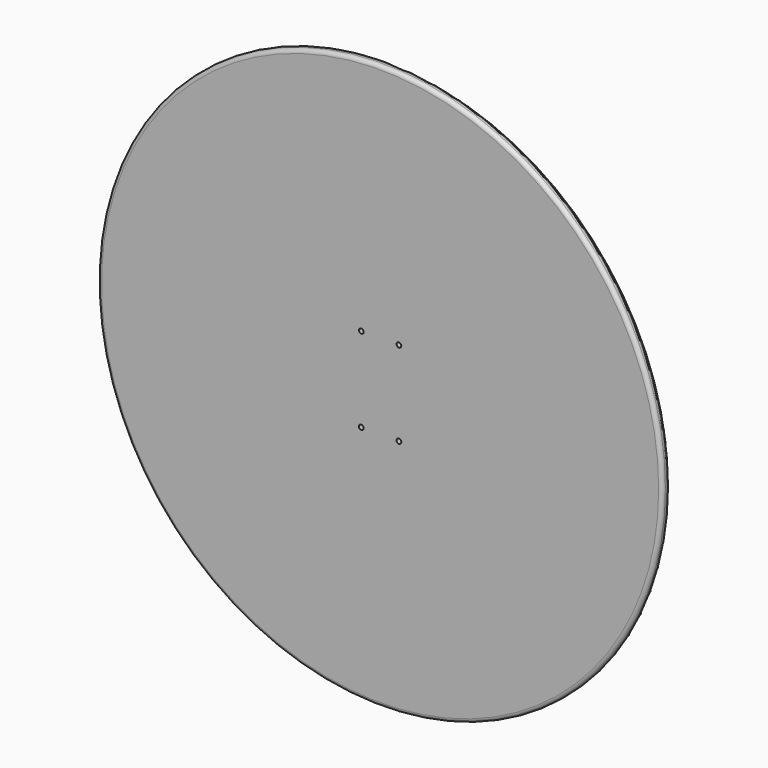
from build123d import *

# Parameters (mm, degrees)
F0_R     = 381
F1_DEPTH = 12.7
F2_R     = 5.08
F3_R     = 3.175
F4_DEPTH = 12.7
F5_R     = 375.92
F6_DEPTH = 2.54
F7_R     = 1.26999
F8_R     = 88.9
F8_R_2   = 50.8
F8_R_3   = 76.2
F9_DEPTH = 12.7
F10_R    = 6.34999


# Not quite as in the source:
# - a fillet or chamfer is up to 0.001 mm smaller than in the source, because OpenCascade refuses the exact size


with BuildPart() as f1:
    # F0 (on Front) → F1 (new body)
    with BuildSketch(Plane.XZ):
        Circle(F0_R)
    extrude(amount=F1_DEPTH)

    # F2
    f2_edges = [f1.edges().sort_by_distance(p)[0] for p in [
        (-381, -12.7, 0),
        (-381, 0, 0),
    ]]
    fillet(f2_edges, radius=F2_R)

    # F3 (on face) → F4 (cut)
    with BuildSketch(Plane.XZ.offset(12.7)):
        with Locations((-25.4, 57.15)):
            Circle(F3_R)
        with Locations((25.4, 57.15)):
            Circle(F3_R)
        with Locations((-25.4, -57.15)):
            Circle(F3_R)
        with Locations((25.4, -57.15)):
            Circle(F3_R)
    extrude(amount=-F4_DEPTH, mode=Mode.SUBTRACT)

    # F5 (on face) → F6 (join)
    with BuildSketch(Plane(origin=(0, 0, 0), x_dir=(-1, 0, 0), z_dir=(0, 1, 0))):
        Circle(F5_R)
        with BuildLine():
            ThreePointArc((13.8301810917, 323.3988637204), (233.7251076258, 223.943459449), (323.6944530953, 0))
            ThreePointArc((323.6944530953, 0), (228.8865428162, -228.8865428162), (0, -323.6944530953))
            ThreePointArc((0, -323.6944530953), (-297.0398470602, -128.6290333601), (-236.0741621082, 221.4657737656))
            ThreePointArc((-236.0741621082, 221.4657737656), (-122.2525479548, 299.7205589933), (13.8301810917, 323.3988637204))
        make_face(mode=Mode.SUBTRACT)
        Polygon((-154.4742758485, 183.9868239484), (-236.0741621082, 221.4657737656), (-282.388240099, -93.3703109622), (-140.2126329417, -183.4818201537), (-33.9375066037, -289.7569464917), align=None)
        with BuildLine():
            ThreePointArc((-236.0741621082, 221.4657737656), (-297.0398470602, -128.6290333601), (0, -323.6944530953))
            Line((0, -323.6944530953), (-33.9375066037, -289.7569464917))
            Line((-33.9375066037, -289.7569464917), (-140.2126329417, -183.4818201537))
            Line((-140.2126329417, -183.4818201537), (-282.388240099, -93.3703109622))
            Line((-282.388240099, -93.3703109622), (-236.0741621082, 221.4657737656))
        make_face()
    extrude(amount=F6_DEPTH)

    # F7 (radius 1.27 in the source; OpenCascade refuses exactly that, so slightly less here)
    f7_edges = [f1.edges().sort_by_distance(p)[0] for p in [
        (94.205891, 2.54, -52.885061),
        (-297.039847, 0, 128.629033),
        (195.274219, 0, 202.726299),
        (94.205891, 0, -52.885061),
        (16.968753, 0, -306.7257),
        (-28.575, 0, -57.15),
        (22.225, 0, -57.15),
        (-28.575, 0, 57.15),
        (22.225, 0, 57.15),
    ]]
    fillet(f7_edges, radius=F7_R)

    # F8 (on face) → F9 (join)
    with BuildSketch(Plane(origin=(0, 0, 0), x_dir=(-1, 0, 0), z_dir=(0, 1, 0))):
        with Locations((-223.9369153976, -103.2387167215)):
            Circle(F8_R)
        with Locations((236.2960875034, 19.1194508225)):
            Circle(F8_R_2)
        with Locations((154.5488387346, -124.6951445937)):
            Circle(F8_R_3)
        Polygon((100.0506654382, 276.4718830585), (-60.4161508381, 225.0014096498), (-110.3727966547, 97.8390201926), (0, 168.989405036), (133.3551108837, 75.1314535737), (196.9362944365, 196.2384879589), (50.0940196216, 175.044760108), align=None)
    extrude(amount=F9_DEPTH)

    # F10 (radius 6.35 in the source; OpenCascade refuses exactly that, so slightly less here)
    f10_edges = [f1.edges().sort_by_distance(p)[0] for p in [
        (-66.677555, 12.7, 122.060429),
        (-165.145703, 12.7, 135.684971),
        (55.186398, 12.7, 133.414213),
        (85.394474, 12.7, 161.420215),
        (-165.145703, 0, 135.684971),
        (-66.677555, 0, 122.060429),
        (55.186398, 0, 133.414213),
        (-75.072343, 12.7, 225.758322),
        (-123.515157, 12.7, 185.641624),
        (-19.817257, 12.7, 250.736646),
        (-75.072343, 0, 225.758322),
        (-185.496088, 0, 19.119451),
        (-185.496088, 12.7, 19.119451),
        (-78.348839, 12.7, -124.695145),
        (-78.348839, 0, -124.695145),
        (312.836915, 12.7, -103.238717),
    ]]
    fillet(f10_edges, radius=F10_R)


solid = f1.part
